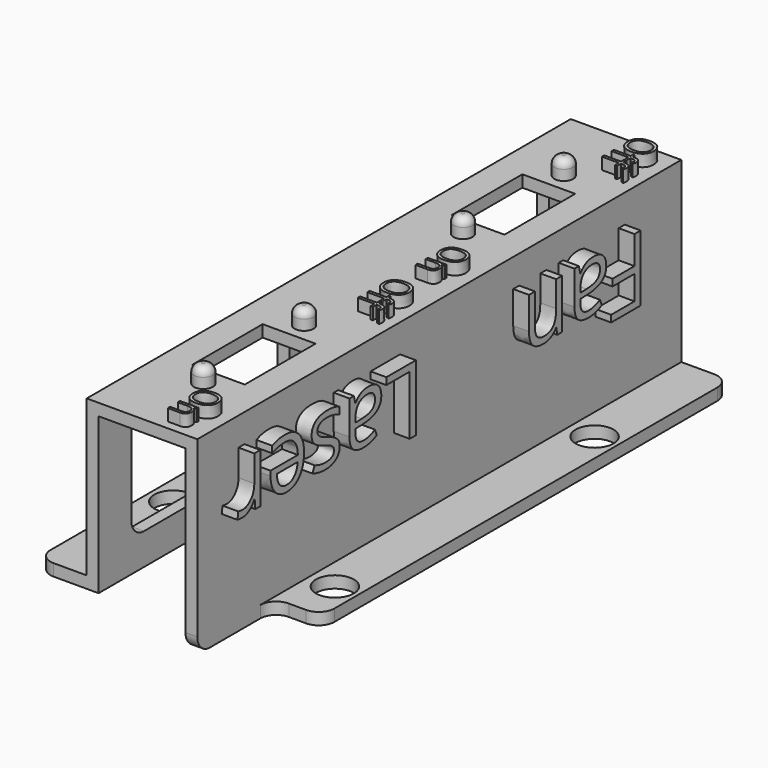
from build123d import *

# Parameters (mm, degrees)
F1_DEPTH        = 76.6
F2_R            = 2.4
F3_DEPTH        = 10
F4_W            = 25
F4_H            = 15
F5_DEPTH        = 1.5
F6_W            = 6.7
F6_H            = 11.2
F7_DEPTH        = 1.5
F8_R            = 1.2
F9_DEPTH        = 2.3
F10_R           = 1
F11_R           = 2
F12_TEXT_SIZE   = 4.4746304435
F12_TEXT_SIZE_2 = 4.3576940536
F13_DEPTH       = 1.5
F14_W           = 6.19
F14_H           = 11.9761225939
F15_DEPTH       = 1.5
F16_TEXT_SIZE   = 11.7185887175
F16_TEXT_SIZE_2 = 11.7180555556
F17_DEPTH       = 2
F18_W           = 11
F18_H           = 1.5
F19_DEPTH       = 22.53
F20_R           = 2


# Not quite as in the source:
# - Text() gives the source's letters only with a copy of the font that has no kerning and outlines rounded to 1/6400 em; it was checked with that copy


with BuildPart() as f1:
    # F0 (on Front) → F1 (new body)
    with BuildSketch(Plane.XZ):
        Polygon((0, 1.5), (0, 0), (7.69, 0), (7.69, 19.73), (18.69, 19.73), (18.69, -2.8), (26.38, -2.8), (26.38, -1.3), (20.19, -1.3), (20.19, 21.23), (6.19, 21.23), (6.19, 1.5), align=None)
    extrude(amount=F1_DEPTH)

    # F2 (on face) → F3 (cut)
    with BuildSketch(Plane.XY.offset(1.5)):
        with Locations((3, -17.82)):
            Circle(F2_R)
        with Locations((3, -58.92)):
            Circle(F2_R)
        with Locations((23.4651640058, -58.92)):
            Circle(F2_R)
        with Locations((23.4651640058, -17.82)):
            Circle(F2_R)
    extrude(amount=-F3_DEPTH, mode=Mode.SUBTRACT)

    # F4 (on face) → F5 (cut, through all)
    with BuildSketch(Plane(origin=(6.19, 0, 0), x_dir=(0, -1, 0), z_dir=(-1, 0, 0))):
        with Locations((17.82, 11.5)):
            Rectangle(F4_W, F4_H)
        with Locations((58.92, 11.5)):
            Rectangle(F4_W, F4_H)
    extrude(amount=-F5_DEPTH, mode=Mode.SUBTRACT)

    # F6 (on face) → F7 (cut, through all)
    with BuildSketch(Plane.XY.offset(21.23)):
        with Locations((13.19, -17.82)):
            Rectangle(F6_W, F6_H)
        with Locations((13.19, -58.92)):
            Rectangle(F6_W, F6_H)
    extrude(amount=-F7_DEPTH, mode=Mode.SUBTRACT)

    # F8 (on face) → F9 (join)
    with BuildSketch(Plane.XY.offset(21.23)):
        with Locations((13.19, -9.85)):
            Circle(F8_R)
        with Locations((13.19, -25.79)):
            Circle(F8_R)
        with Locations((13.19, -50.95)):
            Circle(F8_R)
        with Locations((13.19, -66.89)):
            Circle(F8_R)
    extrude(amount=F9_DEPTH)

    # F10
    f10_edges = [f1.edges().sort_by_distance(p)[0] for p in [
        (11.99, -9.85, 23.53),
        (11.99, -25.79, 23.53),
        (11.99, -50.95, 23.53),
        (11.99, -66.89, 23.53),
    ]]
    fillet(f10_edges, radius=F10_R)

    # F11
    f11_edges = [f1.edges().sort_by_distance(p)[0] for p in [
        (6.94, -5.32, 4),
        (6.94, -5.32, 19),
        (6.94, -30.32, 19),
        (6.94, -30.32, 4),
        (6.94, -46.42, 19),
        (6.94, -46.42, 4),
        (6.94, -71.42, 19),
        (6.94, -71.42, 4),
    ]]
    fillet(f11_edges, radius=F11_R)

    # F12 (on face) → F13 (join)
    with BuildSketch(Plane.XY.offset(21.23)):
        with Locations(Location((15.4580594707, -39.4219394555), (0, 0, -90))):
            Text('Off', F12_TEXT_SIZE, font='Open Sans', text_align=(TextAlign.LEFT, TextAlign.BOTTOM))
        with Locations(Location((15.5422536715, -69.7456515782), (0, 0, -90))):
            Text('On', F12_TEXT_SIZE_2, font='Open Sans', text_align=(TextAlign.LEFT, TextAlign.BOTTOM))
        with Locations(Location((15.4395983974, -0.7480261847), (0, 0, -90))):
            Text('Off', F12_TEXT_SIZE, font='Open Sans', text_align=(TextAlign.LEFT, TextAlign.BOTTOM))
        with Locations(Location((15.5237925981, -30.5067803711), (0, 0, -90))):
            Text('On', F12_TEXT_SIZE_2, font='Open Sans', text_align=(TextAlign.LEFT, TextAlign.BOTTOM))
    extrude(amount=F13_DEPTH)

    # F14 (on face) → F15 (cut, through all)
    with BuildSketch(Plane.XY.offset(-1.3)):
        with Locations((23.285, -70.6119387031)):
            Rectangle(F14_W, F14_H)
    extrude(amount=-F15_DEPTH, mode=Mode.SUBTRACT)

    # F16 (on face) → F17 (join)
    with BuildSketch(Plane.YZ.offset(20.19)):
        with Locations(Location((-7.7845625948, 17.6460508974), (0, 0, 180))):
            Text('Fan', F16_TEXT_SIZE, font='Open Sans', text_align=(TextAlign.LEFT, TextAlign.BOTTOM))
        with Locations(Location((-43.358267812, 17.6456670208), (0, 0, 180))):
            Text('Laser', F16_TEXT_SIZE_2, font='Open Sans', text_align=(TextAlign.LEFT, TextAlign.BOTTOM))
    extrude(amount=F17_DEPTH)

    # F18 (on face) → F19 (join)
    with BuildSketch(Plane(origin=(0, 0, 19.73), x_dir=(1, 0, 0), z_dir=(0, 0, -1))):
        with Locations((13.19, 0.75)):
            Rectangle(F18_W, F18_H)
    extrude(amount=F19_DEPTH)

    # F20
    f20_edges = [f1.edges().sort_by_distance(p)[0] for p in [
        (26.38, 0, -2.05),
        (0, 0, 0.75),
        (0, -76.6, 0.75),
        (26.38, -64.623877, -2.05),
        (20.19, -64.623877, -2.05),
        (19.44, -76.6, -2.8),
    ]]
    fillet(f20_edges, radius=F20_R)


solid = f1.part
